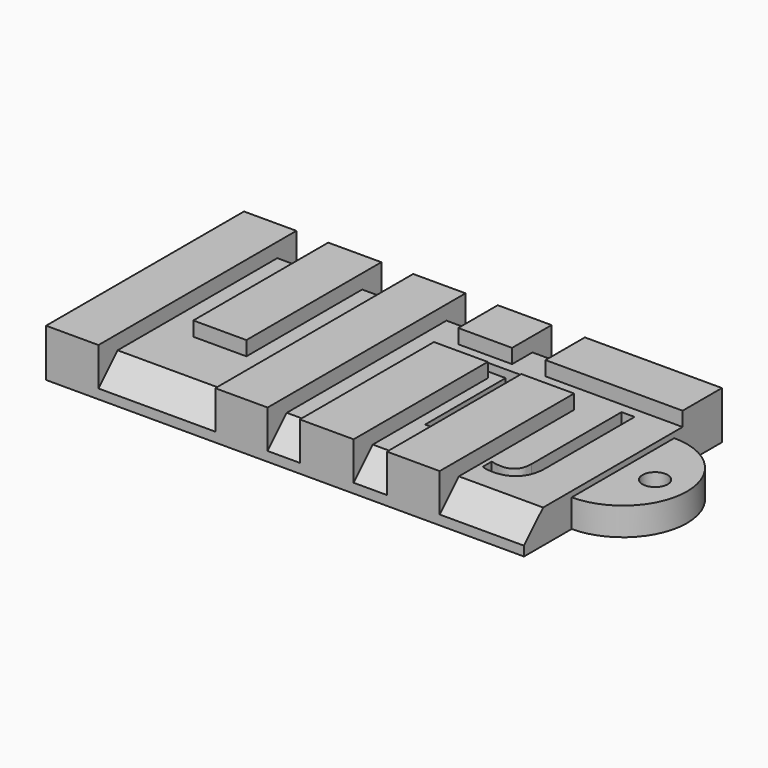
from build123d import *

# Parameters (mm, degrees)
F1_DEPTH     = 4.2
F0_W         = 6.5777550638
F0_H         = 31.0568130806
F0_W_2       = 6.6643171012
F0_H_2       = 21.1724707555
F0_W_3       = 6.5723955631
F0_W_4       = 6.7562386394
F0_H_3       = 6.1960610162
F0_H_4       = 21.0460054386
F0_W_5       = 6.6203959286
F0_H_5       = 21.0919662077
F0_W_6       = 17.2071668506
F0_H_6       = 6.1697455656
F2_DEPTH     = 6
F0_R         = 1.5875
F3_DEPTH     = 3.5
F4_TEXT_SIZE = 19.7454847188
F5_DEPTH     = 25
F6_SIZE      = 3


# Not quite as in the source:
# - Text() gives the source's letters only with a copy of the font that has no kerning and outlines rounded to 1/6400 em; it was checked with that copy


with BuildPart() as f1:
    # F0 (on Top) → F1 (new body)
    with BuildSketch(Plane.XY):
        Polygon((-63.7559369206, -7.0417550277), (-67.7545294166, -7.0417550277), (-67.7545294166, -38.0985681083), (-53.0930310488, -38.0985681083), (-53.0930310488, -7.0417550277), (-57.0916198194, -7.0417550277), (-57.0916198194, -28.2142257832), (-63.7559369206, -28.2142257832), align=None)
    extrude(amount=F1_DEPTH)



with BuildPart() as f1b:
    # F0 (on Top) → F1, piece 2 (new body)
    with BuildSketch(Plane.XY):
        Polygon((-46.5206354856, -7.0417550277), (-46.5206354856, -38.0985681083), (-42.4760840833, -38.0985681083), (-42.4760840833, -17.0525626697), (-35.719845444, -17.0525626697), (-35.719845444, -38.0985681083), (-31.5394513309, -38.0985681083), (-31.5394513309, -17.0066019006), (-24.9190554023, -17.0066019006), (-24.9190554023, -38.0985681083), (-14.3322844803, -38.0985681083), (-14.3322844803, -30.6171796859), (-14.3322844803, -14.5231434501), (-14.3322844803, -13.2115005933), (-31.5394513309, -13.2115005933), (-31.5394513309, -7.0417550277), (-35.719845444, -7.0417550277), (-35.719845444, -13.2378160439), (-42.4760840833, -13.2378160439), (-42.4760840833, -7.0417550277), align=None)
    extrude(amount=F1_DEPTH)


with BuildPart() as f1_1:
    add(f1.part)

    add(f1b.part)  # F2 merges F1b
    # F0 (on Top) → F2 (join)
    with BuildSketch(Plane.XY):
        with Locations((-71.0434069484, -22.570161568)):
            Rectangle(F0_W, F0_H)
        with Locations((-60.42377837, -17.6279904054)):
            Rectangle(F0_W_2, F0_H_2)
        with Locations((-49.8068332672, -22.570161568)):
            Rectangle(F0_W_3, F0_H)
        with Locations((-39.0979647636, -10.1397855358)):
            Rectangle(F0_W_4, F0_H_3)
        with Locations((-39.0979647636, -27.575565389)):
            Rectangle(F0_W_4, F0_H_4)
        with Locations((-28.2292533666, -27.5525850045)):
            Rectangle(F0_W_5, F0_H_5)
        with Locations((-22.9358679056, -10.1266278105)):
            Rectangle(F0_W_6, F0_H_6)
    extrude(amount=F2_DEPTH)

    # F0 (on Top) → F3 (join)
    with BuildSketch(Plane.XY):
        with BuildLine():
            Line((-14.3322844803, -14.5231434501), (-14.3322844803, -30.6171796859))
            ThreePointArc((-14.3322844803, -30.6171796859), (-6.2852663624, -22.570161568), (-14.3322844803, -14.5231434501))
        make_face()
        with Locations((-10.300190188, -22.570161568)):
            Circle(F0_R, mode=Mode.SUBTRACT)
    extrude(amount=F3_DEPTH)

    # F4 (on face) → F5 (cut)
    with BuildSketch(Plane.XY.offset(4.2)):
        with Locations((-39.0060693026, -28.5764010325)):
            Text('T', F4_TEXT_SIZE, font='Open Sans', text_align=(TextAlign.LEFT, TextAlign.BOTTOM))
        with Locations((-22.8147171438, -28.5764010325)):
            Text('J', F4_TEXT_SIZE, font='Open Sans', text_align=(TextAlign.LEFT, TextAlign.BOTTOM))
    extrude(amount=-F5_DEPTH, mode=Mode.SUBTRACT)

    # F6
    f6_edges = [f1_1.edges().sort_by_distance(p)[0] for p in [
        (-65.755233, -7.041755, 4.2),
        (-55.092325, -7.041755, 4.2),
        (-44.49836, -7.041755, 4.2),
        (-33.629648, -7.041755, 4.2),
        (-60.42378, -38.098568, 4.2),
        (-44.49836, -38.098568, 4.2),
        (-33.629648, -38.098568, 4.2),
        (-19.62567, -38.098568, 4.2),
    ]]
    chamfer(f6_edges, length=F6_SIZE)


solid = f1_1.part
